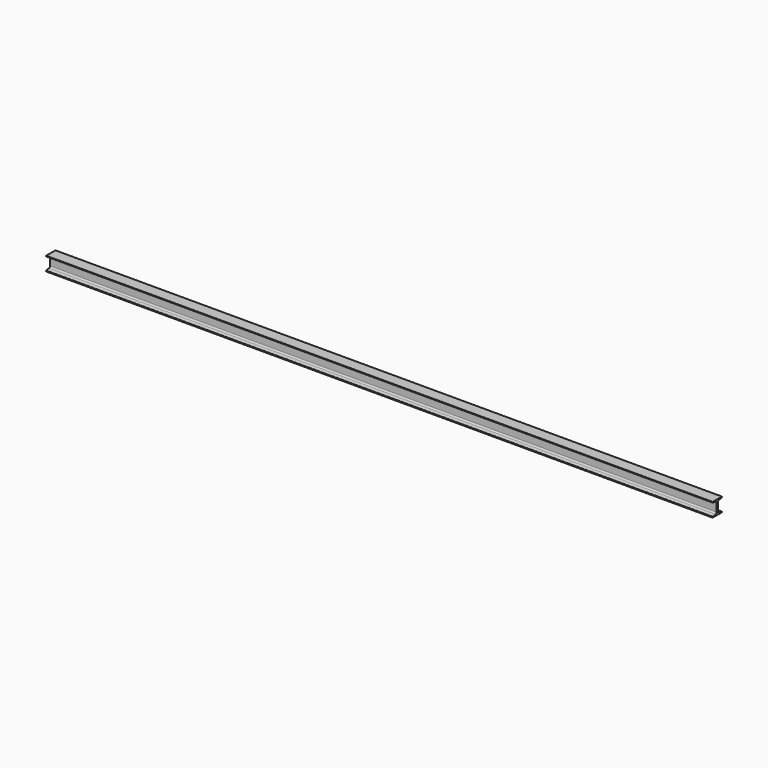
from build123d import *

# Parameters (mm, degrees)
F1_DEPTH = 1828.8


# Not quite as in the source:
# - ends of sketch curves that miss each other by under 0.0002 mm in the source are joined


with BuildPart() as f1:
    # F0 (on Right) → F1 (new body, symmetric)
    with BuildSketch(Plane.YZ):
        with BuildLine():
            ThreePointArc((29.8166013588, 33.5523159732), (31.2936627946, 34.4050969282), (31.877, 36.007802))
            Line((31.877, 36.007802), (31.877, 38.1))
            Line((31.877, 38.1), (-31.877, 38.1))
            Line((-31.877, 38.1), (-31.877, 36.007802))
            ThreePointArc((-31.877, 36.007802), (-31.2936627946, 34.4050969282), (-29.8166013588, 33.5523159732))
            Line((-29.8166013588, 33.5523159732), (-11.1795814, 30.2661066))
            ThreePointArc((-11.1795814, 30.2661066), (-6.3425799325, 27.4734582433), (-4.4323, 22.225))
            Line((-4.4323, 22.225), (-4.4323, -22.225))
            ThreePointArc((-4.4323, -22.225), (-6.3425799325, -27.4734582433), (-11.1795807041, -30.2661105468))
            Line((-11.1795807041, -30.2661105468), (-29.8166028, -33.5523078))
            ThreePointArc((-29.8166028, -33.5523078), (-31.2936627946, -34.4050969282), (-31.877, -36.007802))
            Line((-31.877, -36.007802), (-31.877, -38.1))
            Line((-31.877, -38.1), (31.877, -38.1))
            Line((31.877, -38.1), (31.877, -36.007802))
            ThreePointArc((31.877, -36.007802), (31.2936627946, -34.4050969282), (29.8166013588, -33.5523159732))
            Line((29.8166013588, -33.5523159732), (11.1795814, -30.2661066))
            ThreePointArc((11.1795814, -30.2661066), (6.3425799325, -27.4734582433), (4.4323, -22.225))
            Line((4.4323, -22.225), (4.4323, 22.225))
            ThreePointArc((4.4323, 22.225), (6.3425799325, 27.4734582433), (11.1795807041, 30.2661105468))
            Line((11.1795807041, 30.2661105468), (29.8166013588, 33.5523159732))
        make_face()
    extrude(amount=F1_DEPTH, both=True)


solid = f1.part
